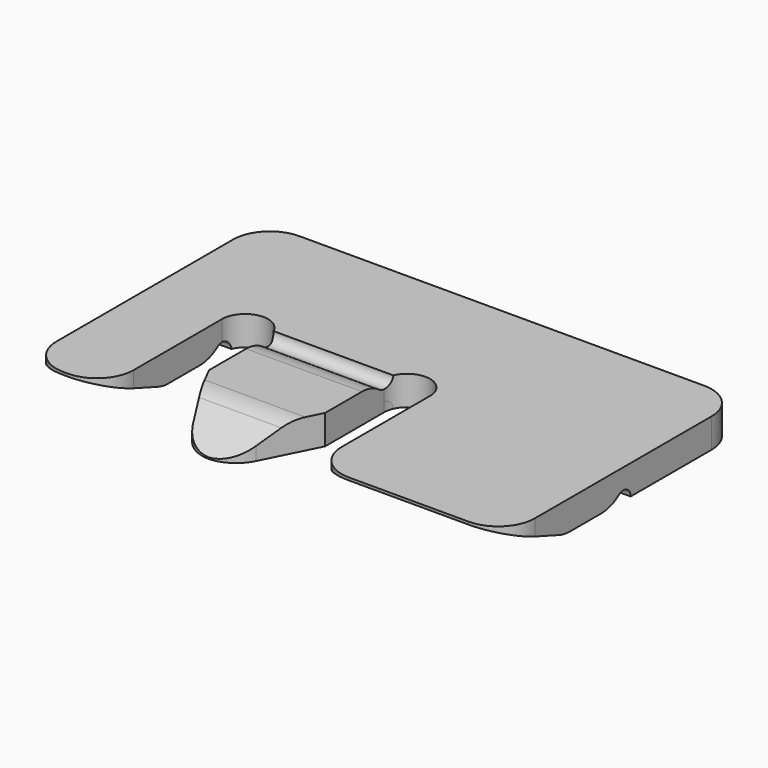
from build123d import *

# Parameters (mm, degrees)
F1_DEPTH      = 4
F3_DEPTH      = 65.001
F5_DEPTH      = 2
F8_DEPTH      = 20
F9_SIZE2      = 6.5817930688
F9_SIZE       = 3.8
F10_SIZE2     = 3.6397023427
F10_SIZE      = 10
F10_2_SIZE2   = 3.6397023427
F10_2_SIZE    = 10
F11_T1_DEPTH  = 19.0305228795
F11_T3_DEPTH  = 14.9081745177
F11_T5_DEPTH  = 30.6581745177
F11_T7_DEPTH  = 38.75
F11_T9_DEPTH  = 23
F11_T11_DEPTH = 28.25
F11_T13_DEPTH = 29
F11_T15_DEPTH = 25.3602976573
F11_T17_DEPTH = 15.6508497187


# Not quite as in the source:
# - a fillet or chamfer that OpenCascade refuses, or shapes differently, is made with other operations: its cross-section is extruded or revolved along the edge and cut away or added


with BuildPart() as f1:
    # F0 (on Top) → F1 (new body)
    with BuildSketch(Plane.XY):
        with BuildLine():
            Line((32.5, -20), (32.5, 20))
            Line((32.5, 20), (-32.5, 20))
            Line((-32.5, 20), (-32.5, -20))
            Line((-32.5, -20), (-22, -20))
            Line((-22, -20), (-22, 0))
            ThreePointArc((-22, 0), (-18.875, 3.125), (-15.75, 0))
            Line((-15.75, 0), (-15.75, -10))
            Line((-15.75, -10), (-10.75, -20))
            Line((-10.75, -20), (-5, -20))
            Line((-5, -20), (0, -10))
            Line((0, -10), (0, 0))
            ThreePointArc((0, 0), (3.125, 3.125), (6.25, 0))
            Line((6.25, 0), (6.25, -20))
            Line((6.25, -20), (32.5, -20))
        make_face()
    extrude(amount=F1_DEPTH)

    # F2 (on face) → F3 (cut, through all)
    with BuildSketch(Plane(origin=(-32.5, 0, 0), x_dir=(0, -1, 0), z_dir=(-1, 0, 0))):
        with BuildLine():
            Line((-1.25, 0), (1.25, 0))
            ThreePointArc((1.25, 0), (0, 1.25), (-1.25, 0))
        make_face()
    extrude(amount=-F3_DEPTH, mode=Mode.SUBTRACT)

    # F4 (on face) → F5 (join)
    with BuildSketch(Plane.XY):
        with BuildLine():
            ThreePointArc((0, 0), (0.0659177721, 0.6384676365), (0.2608901907, 1.25))
            Line((0.2608901907, 1.25), (-16.0108901907, 1.25))
            ThreePointArc((-16.0108901907, 1.25), (-15.8159177721, 0.6384676365), (-15.75, 0))
            Line((-15.75, 0), (-15.75, -1.25))
            Line((-15.75, -1.25), (0, -1.25))
            Line((0, -1.25), (0, 0))
        make_face()
    extrude(amount=F5_DEPTH)

    # F7 (on offset) → F8 (cut)
    with BuildSketch(Plane(origin=(-17.75, 0, 0), x_dir=(0, -1, 0), z_dir=(-1, 0, 0))):
        with BuildLine():
            Line((1.25, 4), (0, 4))
            Line((0, 4), (-1.25, 4))
            ThreePointArc((-1.25, 4), (0, 2.75), (1.25, 4))
        make_face()
    extrude(amount=-F8_DEPTH, mode=Mode.SUBTRACT)

    # F9
    f9_edges = [f1.edges().sort_by_distance(p)[0] for p in [
        (-7.875, -20, 4),
    ]]
    f9_side = f1.faces().sort_by_distance((-7.875, -20, 2))[0]
    chamfer(f9_edges, length=F9_SIZE, length2=F9_SIZE2, reference=f9_side)

    # F10
    f10_edges = [f1.edges().sort_by_distance(p)[0] for p in [
        (-27.25, -20, 0),
    ]]
    f10_side = f1.faces().sort_by_distance((-27.25, -10.625, 0))[0]
    chamfer(f10_edges, length=F10_SIZE, length2=F10_SIZE2, reference=f10_side)

    # F10#2
    f10_2_edges = [f1.edges().sort_by_distance(p)[0] for p in [
        (19.375, -20, 0),
    ]]
    f10_2_side = f1.faces().sort_by_distance((19.375, -10.625, 0))[0]
    chamfer(f10_2_edges, length=F10_2_SIZE, length2=F10_2_SIZE2, reference=f10_2_side)

    # F11: fillet of radius 5 on 14 edges, made by hand

    # F11_s2 → F11_t1 (cut)
    with BuildSketch(Plane.YZ.offset(-17.3902614398)):
        with BuildLine():
            ThreePointArc((-12.0784609691, 4), (-13.3725561946, 3.8296291314), (-14.5784609691, 3.3301270189))
            Line((-14.5784609691, 3.3301270189), (-13.4182069312, 4))
            Line((-13.4182069312, 4), (-12.0784609691, 4))
        make_face()
    extrude(amount=F11_T1_DEPTH, mode=Mode.SUBTRACT)

    # F11_s4 → F11_t3 (cut)
    with BuildSketch(Plane.YZ.offset(-34.7040872589)):
        with BuildLine():
            ThreePointArc((-9.1183650965, 0), (-9.9866059848, 0.0759612349), (-10.8284658131, 0.3015368961))
            Line((-10.8284658131, 0.3015368961), (-10, 0))
            Line((-10, 0), (-9.1183650965, 0))
        make_face()
    extrude(amount=F11_T3_DEPTH, mode=Mode.SUBTRACT)

    # F11_s6 → F11_t5 (cut)
    with BuildSketch(Plane.YZ.offset(4.0459127411)):
        with BuildLine():
            ThreePointArc((-9.1183650965, 0), (-9.9866059848, 0.0759612349), (-10.8284658131, 0.3015368961))
            Line((-10.8284658131, 0.3015368961), (-10, 0))
            Line((-10, 0), (-9.1183650965, 0))
        make_face()
    extrude(amount=F11_T5_DEPTH, mode=Mode.SUBTRACT)

    # F11_s8 → F11_t7 (cut)
    with BuildSketch(Plane.YZ):
        with BuildLine():
            ThreePointArc((-3.75, 0), (-2.1688611699, 0.2565835097), (-0.75, 1))
            ThreePointArc((-0.75, 1), (-1.1180339887, 0.5590169944), (-1.25, 0))
            Line((-1.25, 0), (-3.75, 0))
        make_face()
    extrude(amount=F11_T7_DEPTH, mode=Mode.SUBTRACT)

    # F11_s10 → F11_t9 (cut)
    with BuildSketch(Plane.YZ.offset(-38.75)):
        with BuildLine():
            ThreePointArc((-0.75, 1), (-2.1688611699, 0.2565835097), (-3.75, 0))
            Line((-3.75, 0), (-1.25, 0))
            ThreePointArc((-1.25, 0), (-1.1180339887, 0.5590169944), (-0.75, 1))
        make_face()
    extrude(amount=F11_T9_DEPTH, mode=Mode.SUBTRACT)

    # F11_s12 → F11_t11 (cut)
    with BuildSketch(Plane.YZ.offset(-22)):
        with BuildLine():
            ThreePointArc((-0.75, 3), (-2.1688611699, 3.7434164903), (-3.75, 4))
            Line((-3.75, 4), (-1.25, 4))
            ThreePointArc((-1.25, 4), (-1.1180339887, 3.4409830056), (-0.75, 3))
        make_face()
    extrude(amount=F11_T11_DEPTH, mode=Mode.SUBTRACT)

    # F11_s14 → F11_t13 (cut)
    with BuildSketch(Plane.XY.offset(-12.5)):
        with BuildLine():
            ThreePointArc((-27.5, 20), (-31.0355339059, 18.5355339059), (-32.5, 15))
            Line((-32.5, 15), (-32.5, 20))
            Line((-32.5, 20), (-27.5, 20))
        make_face()
        with BuildLine():
            ThreePointArc((32.5, 15), (31.0355339059, 18.5355339059), (27.5, 20))
            Line((27.5, 20), (32.5, 20))
            Line((32.5, 20), (32.5, 15))
        make_face()
    extrude(amount=F11_T13_DEPTH, mode=Mode.SUBTRACT)

    # F11_s16 → F11_t15 (cut)
    with BuildSketch(Plane.XY.offset(-8.8602976573)):
        with BuildLine():
            ThreePointArc((-32.5, -15), (-31.0355339059, -18.5355339059), (-27.5, -20))
            Line((-27.5, -20), (-32.5, -20))
            Line((-32.5, -20), (-32.5, -15))
        make_face()
        with BuildLine():
            ThreePointArc((-22, -15), (-23.4644660941, -18.5355339059), (-27, -20))
            Line((-27, -20), (-22, -20))
            Line((-22, -20), (-22, -15))
        make_face()
        with BuildLine():
            ThreePointArc((11.25, -20), (7.7144660941, -18.5355339059), (6.25, -15))
            Line((6.25, -15), (6.25, -20))
            Line((6.25, -20), (11.25, -20))
        make_face()
        with BuildLine():
            ThreePointArc((32.5, -15), (31.0355339059, -18.5355339059), (27.5, -20))
            Line((27.5, -20), (32.5, -20))
            Line((32.5, -20), (32.5, -15))
        make_face()
    extrude(amount=F11_T15_DEPTH, mode=Mode.SUBTRACT)

    # F11_s18 → F11_t17 (cut)
    with BuildSketch(Plane.XY.offset(-7.7254248594)):
        with BuildLine():
            ThreePointArc((-8.0901699437, -20), (-5.4615143832, -19.2532540418), (-3.6180339887, -17.2360679775))
            Line((-3.6180339887, -17.2360679775), (-5, -20))
            Line((-5, -20), (-8.0901699437, -20))
        make_face()
        with BuildLine():
            ThreePointArc((-12.1319660113, -17.2360679775), (-10.2884856168, -19.2532540418), (-7.6598300563, -20))
            Line((-7.6598300563, -20), (-10.75, -20))
            Line((-10.75, -20), (-12.1319660113, -17.2360679775))
        make_face()
    extrude(amount=F11_T17_DEPTH, mode=Mode.SUBTRACT)


solid = f1.part
